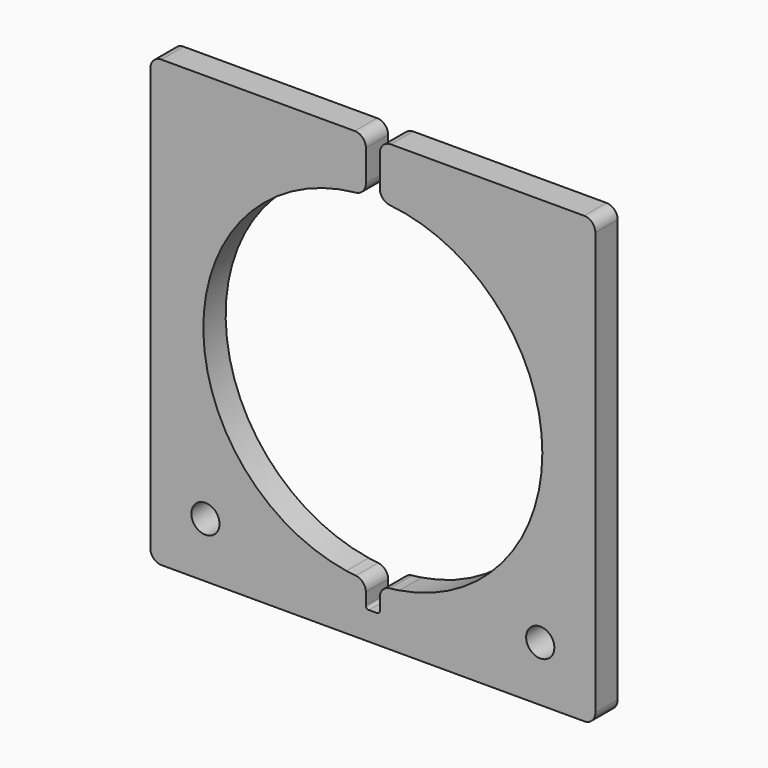
from build123d import *

# Parameters (mm, degrees)
F0_R     = 5.05
F0_W     = 2.5
F0_H     = 10
F1_DEPTH = 10
F2_R     = 4
F3_R     = 1


# Not quite as in the source:
# - a feature names something its author has since deleted; it is built from what else it names


with BuildPart() as f1:
    # F0 (on Front) → F1 (new body)
    with BuildSketch(Plane.XZ):
        with BuildLine():
            Line((-79.75, 79.75), (-79.75, -79.75))
            Line((-79.75, -79.75), (-2.5, -79.75))
            Line((-2.5, -79.75), (-2.5, -69.75))
            Line((-2.5, -69.75), (-2.5, -60.6985378737))
            ThreePointArc((-2.5, -60.6985378737), (-6.0183598459, -60.4511525512), (-9.5164331553, -60))
            ThreePointArc((-9.5164331553, -60), (-60.6476127119, 3.5255598628), (-2.5, 60.6985378737))
            Line((-2.5, 60.6985378737), (-2.5, 79.75))
            Line((-2.5, 79.75), (-79.75, 79.75))
        make_face()
        with Locations((-60, -60)):
            Circle(F0_R, mode=Mode.SUBTRACT)
        with BuildLine():
            Line((2.5, -69.75), (2.5, -79.75))
            Line((2.5, -79.75), (79.75, -79.75))
            Line((79.75, -79.75), (79.75, 79.75))
            Line((79.75, 79.75), (2.5, 79.75))
            Line((2.5, 79.75), (2.5, 60.6985378737))
            ThreePointArc((2.5, 60.6985378737), (43.8317094123, 42.0635679656), (60.75, 0))
            ThreePointArc((60.75, 0), (46.198949199, -39.448949199), (9.5164331553, -60))
            ThreePointArc((9.5164331553, -60), (6.0183598459, -60.4511525512), (2.5, -60.6985378737))
            Line((2.5, -60.6985378737), (2.5, -69.75))
        make_face()
        with BuildLine():
            ThreePointArc((65.05, -60), (60, -65.05), (54.95, -60))
            ThreePointArc((54.95, -60), (60, -54.95), (65.05, -60))
        make_face(mode=Mode.SUBTRACT)
        with Locations((-1.25, -74.75)):
            Rectangle(F0_W, F0_H)
        with Locations((1.25, -74.75)):
            Rectangle(F0_W, F0_H)
    extrude(amount=F1_DEPTH)

    # F2
    f2_edges = [f1.edges().sort_by_distance(p)[0] for p in [
        (79.75, -5, 79.75),
        (-79.75, -5, 79.75),
        (-79.75, -5, -79.75),
        (79.75, -5, -79.75),
        (-2.5, -5, 60.698538),
        (-2.5, -5, 79.75),
        (2.5, -5, 79.75),
        (2.5, -5, 60.698538),
        (2.5, -5, -60.698538),
        (-2.5, -5, -60.698538),
    ]]
    fillet(f2_edges, radius=F2_R)

    # F3
    f3_edges = [f1.edges().sort_by_distance(p)[0] for p in [
        (-2.5, -5, -69.75),
        (2.5, -5, -69.75),
    ]]
    fillet(f3_edges, radius=F3_R)


solid = f1.part
